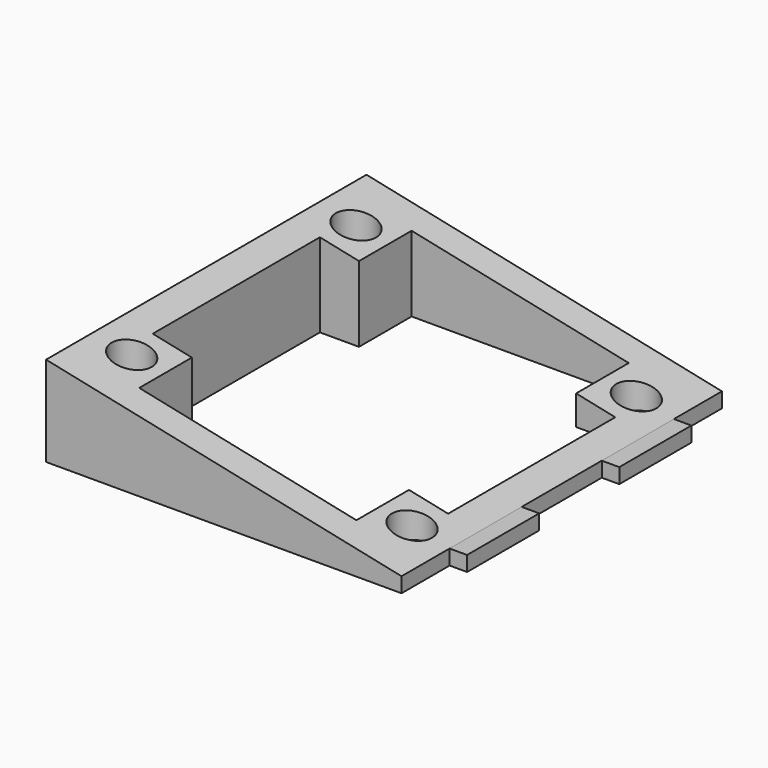
from build123d import *

# Parameters (mm, degrees)
F1_DEPTH = 40
F3_D     = 4
F4_W     = 9
F4_H     = 1.5
F5_DEPTH = 1.75
F6_W     = 9
F6_H     = 1.5
F7_DEPTH = 1.75
F8_W     = 10.8425548855
F8_H     = 10.4324881697
F8_W_2   = 3.9074451145
F8_H_2   = 6.5675118303
F9_DEPTH = 9.001


with BuildPart() as f1:
    # F0 (on Front) → F1 (new body)
    with BuildSketch(Plane.XZ):
        Polygon((0, 9), (0, 0), (35.5, 0), (35.5, 1.5), align=None)
    extrude(amount=F1_DEPTH)

    # F3 (through all)
    with Locations(Plane(origin=(0, 0, 0), x_dir=(1, 0, 0), z_dir=(0, 0, -1))):
        with Locations((3.75, 34), (31.75, 34), (31.75, 6), (3.75, 6)):
            Hole(F3_D / 2)

    # F4 (on face) → F5 (join)
    with BuildSketch(Plane(origin=(0, 0, 0), x_dir=(0, -1, 0), z_dir=(-1, 0, 0))):
        with Locations((29.5, 0.75)):
            Rectangle(F4_W, F4_H)
        with Locations((10.5, 0.75)):
            Rectangle(F4_W, F4_H)
    extrude(amount=F5_DEPTH)

    # F6 (on face) → F7 (join)
    with BuildSketch(Plane.YZ.offset(35.5)):
        with Locations((-10.5, 0.75)):
            Rectangle(F6_W, F6_H)
        with Locations((-29.5, 0.75)):
            Rectangle(F6_W, F6_H)
    extrude(amount=F7_DEPTH)

    # F8 (on face) → F9 (cut, through all)
    with BuildSketch(Plane(origin=(0, 0, 0), x_dir=(1, 0, 0), z_dir=(0, 0, -1))):
        with Locations((23.1712774428, 25.2162440849)):
            Rectangle(F8_W, F8_H)
        with Locations((12.3287225572, 14.7837559151)):
            Rectangle(F8_W, F8_H)
        with Locations((12.3287225572, 25.2162440849)):
            Rectangle(F8_W, F8_H)
        with Locations((23.1712774428, 14.7837559151)):
            Rectangle(F8_W, F8_H)
        with Locations((30.5462774428, 25.2162440849)):
            Rectangle(F8_W_2, F8_H)
        with Locations((30.5462774428, 14.7837559151)):
            Rectangle(F8_W_2, F8_H)
        with Locations((4.9537225572, 14.7837559151)):
            Rectangle(F8_W_2, F8_H)
        with Locations((4.9537225572, 25.2162440849)):
            Rectangle(F8_W_2, F8_H)
        with Locations((12.3287225572, 33.7162440849)):
            Rectangle(F8_W, F8_H_2)
        with Locations((23.1712774428, 33.7162440849)):
            Rectangle(F8_W, F8_H_2)
        with Locations((23.1712774428, 6.2837559151)):
            Rectangle(F8_W, F8_H_2)
        with Locations((12.3287225572, 6.2837559151)):
            Rectangle(F8_W, F8_H_2)
    extrude(amount=-F9_DEPTH, mode=Mode.SUBTRACT)


solid = f1.part
